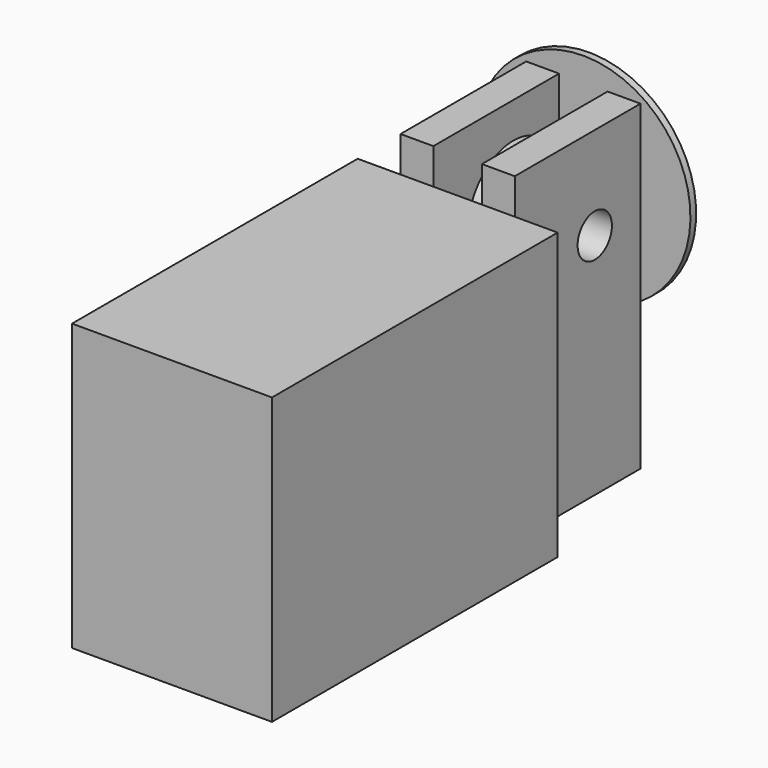
from build123d import *

# Parameters (mm, degrees)
F1_DEPTH  = 11
F3_W      = 3
F3_H      = 20
F3_W_2    = 3.4
F3_H_2    = 10.2
F4_DEPTH  = 25
F5_R      = 1.5
F6_DEPTH  = 25
F5_R_2    = 2.5
F7_DEPTH  = 8
F8_SIZE   = 1.49999
F9_SIZE   = 1.49999
F10_R     = 7.5
F12_DEPTH = 0.5


# Not quite as in the source:
# - a fillet or chamfer is up to 0.001 mm smaller than in the source, because OpenCascade refuses the exact size


with BuildPart() as f1:
    # F0 (on Front) → F1 (new body)
    with BuildSketch(Plane.XZ):
        Polygon((-4, 0), (0, 0), (0, 9.8), (-1.7, 9.8), (-1.7, 22.5), (-4, 22.5), align=None)
    extrude(amount=F1_DEPTH)

    # F2: F1 across face


with BuildPart() as f1_1:
    add(f1.part)
    add(f1.part.mirror(Plane(origin=(0, -5.5, 4.9), x_dir=(0, 1, 0), z_dir=(1, 0, 0))))

    # F3 (on face) → F4 (join)
    with BuildSketch(Plane.XZ.offset(11)):
        with Locations((5.5, 10)):
            Rectangle(F3_W, F3_H)
        with Locations((0, 14.9)):
            Rectangle(F3_W_2, F3_H_2)
        Polygon((-4, 0), (0, 0), (4, 0), (4, 20), (1.7, 20), (1.7, 9.8), (-1.7, 9.8), (-1.7, 20), (-4, 20), align=None)
        with Locations((-5.5, 10)):
            Rectangle(F3_W, F3_H)
    extrude(amount=F4_DEPTH)

    # F5 (on face) → F6 (cut)
    with BuildSketch(Plane.YZ.offset(4)):
        with Locations((-4, 16)):
            Circle(F5_R)
    extrude(amount=-F6_DEPTH, mode=Mode.SUBTRACT)

    # F5 (on face) → F7 (join, through all)
    with BuildSketch(Plane.YZ.offset(4)):
        with Locations((-4, 16)):
            Circle(F5_R_2)
        with Locations((-4, 16)):
            Circle(F5_R, mode=Mode.SUBTRACT)
    extrude(amount=-F7_DEPTH)

    # F8 (size 1.5 in the source; OpenCascade refuses exactly that, so slightly less here)
    f8_edges = [f1_1.edges().sort_by_distance(p)[0] for p in [
        (-1.7, -6.5, 16),
    ]]
    chamfer(f8_edges, length=F8_SIZE)

    # F9 (size 1.5 in the source; OpenCascade refuses exactly that, so slightly less here)
    f9_edges = [f1_1.edges().sort_by_distance(p)[0] for p in [
        (1.7, -6.5, 16),
    ]]
    chamfer(f9_edges, length=F9_SIZE)

    # F10 (on face) → F12 (join)
    with BuildSketch(Plane(origin=(0, 0, 0), x_dir=(-1, 0, 0), z_dir=(0, 1, 0))):
        with Locations((0, 16.6603474262)):
            Circle(F10_R)
    extrude(amount=F12_DEPTH)


solid = f1_1.part
